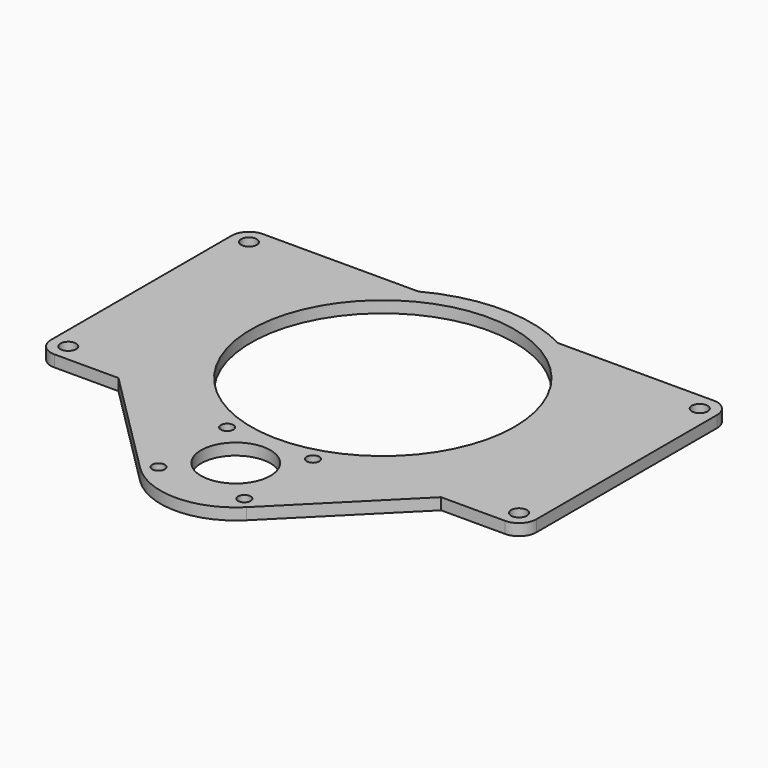
from build123d import *

# Parameters (mm, degrees)
F0_R     = 1.7272
F0_R_2   = 2.15265
F0_R_3   = 9.525
F0_R_4   = 36.195
F1_DEPTH = 3.175
F2_R     = 4.7625


with BuildPart() as f1:
    # F0 (on Top) → F1 (new body)
    with BuildSketch(Plane.XY):
        with BuildLine():
            Line((-19.1686927371, 36.195), (-66.6623, 36.195))
            Line((-66.6623, 36.195), (-66.6623, -35.3695))
            Line((-66.6623, -35.3695), (-44.2988323935, -35.3695))
            Line((-44.2988323935, -35.3695), (-14.5929161967, -65.0754161967))
            ThreePointArc((-14.5929161967, -65.0754161967), (0, -71.12), (14.5929161967, -65.0754161967))
            Line((14.5929161967, -65.0754161967), (44.2988323935, -35.3695))
            Line((44.2988323935, -35.3695), (66.6623, -35.3695))
            Line((66.6623, -35.3695), (66.6623, 36.195))
            Line((66.6623, 36.195), (19.1686927371, 36.195))
            ThreePointArc((19.1686927371, 36.195), (0, 40.9575), (-19.1686927371, 36.195))
        make_face()
        with Locations((-11.7865861589, -62.2690861589)):
            Circle(F0_R, mode=Mode.SUBTRACT)
        with Locations((-61.8998, -30.607)):
            Circle(F0_R_2, mode=Mode.SUBTRACT)
        with Locations((-11.7865861589, -38.6959138411)):
            Circle(F0_R, mode=Mode.SUBTRACT)
        with Locations((11.7865861589, -62.2690861589)):
            Circle(F0_R, mode=Mode.SUBTRACT)
        with Locations((0, -50.4825)):
            Circle(F0_R_3, mode=Mode.SUBTRACT)
        with Locations((11.7865861589, -38.6959138411)):
            Circle(F0_R, mode=Mode.SUBTRACT)
        with Locations((61.8998, -30.607)):
            Circle(F0_R_2, mode=Mode.SUBTRACT)
        with Locations((-61.8998, 31.4325)):
            Circle(F0_R_2, mode=Mode.SUBTRACT)
        Circle(F0_R_4, mode=Mode.SUBTRACT)
        with Locations((61.8998, 31.4325)):
            Circle(F0_R_2, mode=Mode.SUBTRACT)
    extrude(amount=F1_DEPTH)

    # F2
    f2_edges = [f1.edges().sort_by_distance(p)[0] for p in [
        (66.6623, -35.3695, 1.5875),
        (-66.6623, -35.3695, 1.5875),
        (66.6623, 36.195, 1.5875),
        (-66.6623, 36.195, 1.5875),
    ]]
    fillet(f2_edges, radius=F2_R)


solid = f1.part
